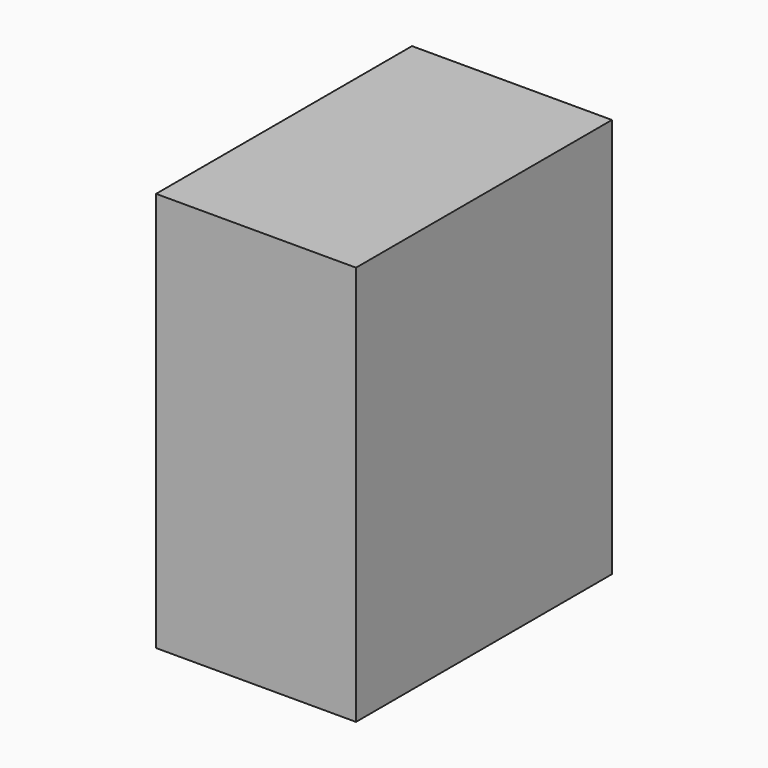
from build123d import *

# Parameters (mm, degrees)
F0_W     = 15.875
F0_H     = 31.75
F1_DEPTH = 25.4


# Not quite as in the source:
# - a feature names something its author has since deleted; it is built from what else it names


with BuildPart() as f1:
    # F0 (on Front) → F1 (new body)
    with BuildSketch(Plane.XZ):
        with Locations((7.9375, -15.875)):
            Rectangle(F0_W, F0_H)
    extrude(amount=F1_DEPTH)


solid = f1.part
